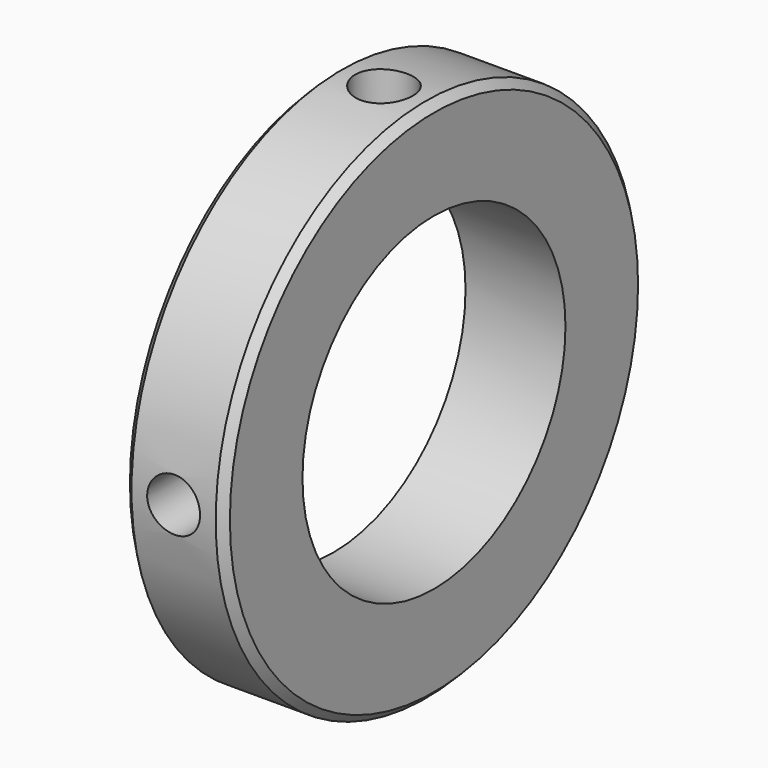
from build123d import *

# Parameters (mm, degrees)
F0_R     = 25.4
F0_R_2   = 15.875
F1_DEPTH = 9.652
F2_SIZE  = 0.762
F7_SIZE  = 0.762
F8_D     = 5.55752
F8_DEPTH = 16.51
F8_TIP   = 1.6696474537
F9_D     = 5.1054
F9_DEPTH = 16.51
F9_TIP   = 1.5338169022


with BuildPart() as f1:
    # F0 (on Right) → F1 (new body)
    with BuildSketch(Plane.YZ):
        Circle(F0_R)
        Circle(F0_R_2, mode=Mode.SUBTRACT)
    extrude(amount=F1_DEPTH)

    # F2
    f2_edges = [f1.edges().sort_by_distance(p)[0] for p in [
        (9.652, -25.4, 0),
    ]]
    chamfer(f2_edges, length=F2_SIZE)

    # F7
    f7_edges = [f1.edges().sort_by_distance(p)[0] for p in [
        (0, -25.4, 0),
    ]]
    chamfer(f7_edges, length=F7_SIZE)

    # F8
    with Locations(Plane.XY.offset(25.4)):
        with Locations((4.826, 0)):
            Hole(F8_D / 2, depth=F8_DEPTH)
            with Locations((0, 0, -(F8_DEPTH + F8_TIP / 2))):  # 118° drill point
                Cone(0, F8_D / 2, F8_TIP, mode=Mode.SUBTRACT)

    # F9
    with Locations(Plane.XZ.offset(25.4)):
        with Locations((4.826, 0)):
            Hole(F9_D / 2, depth=F9_DEPTH)
            with Locations((0, 0, -(F9_DEPTH + F9_TIP / 2))):  # 118° drill point
                Cone(0, F9_D / 2, F9_TIP, mode=Mode.SUBTRACT)


solid = f1.part
